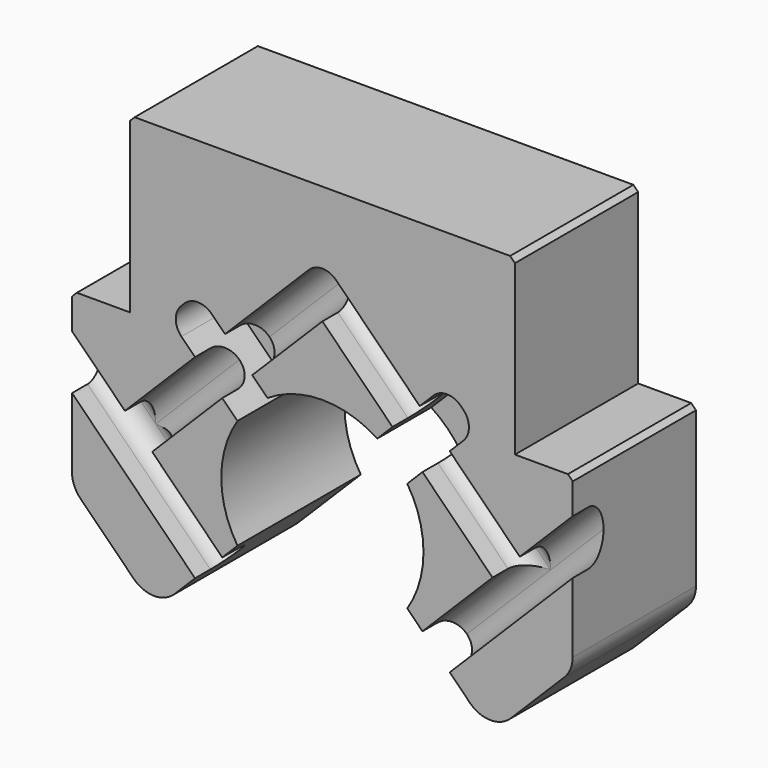
from build123d import *

# Parameters (mm, degrees)
F1_DEPTH = 16
F2_DEPTH = 7
F3_DEPTH = 4
F4_R     = 2
F5_R     = 1.9999
F6_R     = 3
F7_SIZE  = 0.5


# Not quite as in the source:
# - a fillet or chamfer is up to 0.001 mm smaller than in the source, because OpenCascade refuses the exact size
# - a feature names something its author has since deleted; it is built from what else it names


with BuildPart() as f1:
    # F0 (on Front) → F1 (new body)
    with BuildSketch(Plane.XZ):
        with BuildLine():
            ThreePointArc((-5.7041860158, 8.815455853), (0, 10.5), (5.7041860158, 8.815455853))
            Line((5.7041860158, 8.815455853), (7.2831998462, 10.3944696834))
            Line((7.2831998462, 10.3944696834), (0, 17.6776695297))
            Line((0, 17.6776695297), (-7.2831998462, 10.3944696834))
            Line((-7.2831998462, 10.3944696834), (-5.7041860158, 8.815455853))
        make_face()
        with BuildLine():
            ThreePointArc((-8.815455853, 5.7041860158), (-7.4246212025, 7.4246212025), (-5.7041860158, 8.815455853))
            Line((-5.7041860158, 8.815455853), (-7.2831998462, 10.3944696834))
            Line((-7.2831998462, 10.3944696834), (-10.3944696834, 7.2831998462))
            Line((-10.3944696834, 7.2831998462), (-8.815455853, 5.7041860158))
        make_face()
        with BuildLine():
            ThreePointArc((-8.815455853, -5.7041860158), (-10.5, 0), (-8.815455853, 5.7041860158))
            Line((-8.815455853, 5.7041860158), (-10.3944696834, 7.2831998462))
            Line((-10.3944696834, 7.2831998462), (-17.6776695297, 0))
            Line((-17.6776695297, 0), (-10.3944696834, -7.2831998462))
            Line((-10.3944696834, -7.2831998462), (-8.815455853, -5.7041860158))
        make_face()
        with BuildLine():
            ThreePointArc((5.7041860158, 8.815455853), (7.4246212025, 7.4246212025), (8.815455853, 5.7041860158))
            Line((8.815455853, 5.7041860158), (10.3944696834, 7.2831998462))
            Line((10.3944696834, 7.2831998462), (7.2831998462, 10.3944696834))
            Line((7.2831998462, 10.3944696834), (5.7041860158, 8.815455853))
        make_face()
        Polygon((0, 17.6776695297), (7.2831998462, 10.3944696834), (10.111626971, 13.2228968082), (0, 23.3345237792), (-10.111626971, 13.2228968082), (-7.2831998462, 10.3944696834), align=None)
        Polygon((7.2831998462, 10.3944696834), (10.3944696834, 7.2831998462), (13.2228968082, 10.111626971), (10.111626971, 13.2228968082), align=None)
        Polygon((-10.3944696834, 7.2831998462), (-7.2831998462, 10.3944696834), (-10.111626971, 13.2228968082), (-13.2228968082, 10.111626971), align=None)
        Polygon((-17.6776695297, 0), (-10.3944696834, 7.2831998462), (-13.2228968082, 10.111626971), (-20.5060966544, 2.8284271247), (-26, 8.3223304703), (-26, 2.6654762208), (-13.2228968082, -10.111626971), (-10.3944696834, -7.2831998462), align=None)
        Polygon((-13.2228968082, 10.111626971), (-10.111626971, 13.2228968082), (-12.9400540957, 16.0513239329), (-16.0513239329, 12.9400540957), align=None)
        Polygon((17.6776695297, 0), (10.3944696834, -7.2831998462), (13.2228968082, -10.111626971), (26, 2.6654762208), (26, 8.3223304703), (20.5060966544, 2.8284271247), (13.2228968082, 10.111626971), (10.3944696834, 7.2831998462), align=None)
        with BuildLine():
            ThreePointArc((8.815455853, 5.7041860158), (10.5, 0), (8.815455853, -5.7041860158))
            Line((8.815455853, -5.7041860158), (10.3944696834, -7.2831998462))
            Line((10.3944696834, -7.2831998462), (17.6776695297, 0))
            Line((17.6776695297, 0), (10.3944696834, 7.2831998462))
            Line((10.3944696834, 7.2831998462), (8.815455853, 5.7041860158))
        make_face()
        Polygon((16.0513239329, 12.9400540957), (13.2228968082, 10.111626971), (20.5060966544, 2.8284271247), (26, 8.3223304703), (26, 12), (20, 12), (20, 30), (0, 30), (-20, 30), (-20, 12), (-26, 12), (-26, 8.3223304703), (-20.5060966544, 2.8284271247), (-13.2228968082, 10.111626971), (-16.0513239329, 12.9400540957), (-12.9400540957, 16.0513239329), (-10.111626971, 13.2228968082), (0, 23.3345237792), (10.111626971, 13.2228968082), (12.9400540957, 16.0513239329), align=None)
        Polygon((10.111626971, 13.2228968082), (13.2228968082, 10.111626971), (16.0513239329, 12.9400540957), (12.9400540957, 16.0513239329), align=None)
        Polygon((26, 2.6654762208), (13.2228968082, -10.111626971), (17.4655374953, -14.3542676581), (26, -5.8198051534), align=None)
        Polygon((-17.4655374953, -14.3542676581), (-13.2228968082, -10.111626971), (-26, 2.6654762208), (-26, -5.8198051534), align=None)
    extrude(amount=-F1_DEPTH)

    # F0 (on Front) → F2 (cut)
    with BuildSketch(Plane.XZ):
        Polygon((10.111626971, 13.2228968082), (13.2228968082, 10.111626971), (16.0513239329, 12.9400540957), (12.9400540957, 16.0513239329), align=None)
        Polygon((7.2831998462, 10.3944696834), (10.3944696834, 7.2831998462), (13.2228968082, 10.111626971), (10.111626971, 13.2228968082), align=None)
        with BuildLine():
            ThreePointArc((5.7041860158, 8.815455853), (7.4246212025, 7.4246212025), (8.815455853, 5.7041860158))
            Line((8.815455853, 5.7041860158), (10.3944696834, 7.2831998462))
            Line((10.3944696834, 7.2831998462), (7.2831998462, 10.3944696834))
            Line((7.2831998462, 10.3944696834), (5.7041860158, 8.815455853))
        make_face()
        with BuildLine():
            ThreePointArc((-8.815455853, 5.7041860158), (-7.4246212025, 7.4246212025), (-5.7041860158, 8.815455853))
            Line((-5.7041860158, 8.815455853), (-7.2831998462, 10.3944696834))
            Line((-7.2831998462, 10.3944696834), (-10.3944696834, 7.2831998462))
            Line((-10.3944696834, 7.2831998462), (-8.815455853, 5.7041860158))
        make_face()
        Polygon((-13.2228968082, 10.111626971), (-10.111626971, 13.2228968082), (-12.9400540957, 16.0513239329), (-16.0513239329, 12.9400540957), align=None)
        Polygon((-10.3944696834, 7.2831998462), (-7.2831998462, 10.3944696834), (-10.111626971, 13.2228968082), (-13.2228968082, 10.111626971), align=None)
    extrude(amount=-F2_DEPTH, mode=Mode.SUBTRACT)

    # F0 (on Front) → F3 (cut)
    with BuildSketch(Plane.XZ):
        Polygon((0, 17.6776695297), (7.2831998462, 10.3944696834), (10.111626971, 13.2228968082), (0, 23.3345237792), (-10.111626971, 13.2228968082), (-7.2831998462, 10.3944696834), align=None)
        Polygon((17.6776695297, 0), (10.3944696834, -7.2831998462), (13.2228968082, -10.111626971), (26, 2.6654762208), (26, 8.3223304703), (20.5060966544, 2.8284271247), (13.2228968082, 10.111626971), (10.3944696834, 7.2831998462), align=None)
        Polygon((-17.6776695297, 0), (-10.3944696834, 7.2831998462), (-13.2228968082, 10.111626971), (-20.5060966544, 2.8284271247), (-26, 8.3223304703), (-26, 2.6654762208), (-13.2228968082, -10.111626971), (-10.3944696834, -7.2831998462), align=None)
    extrude(amount=-F3_DEPTH, mode=Mode.SUBTRACT)

    # F4
    f4_edges = [f1.edges().sort_by_distance(p)[0] for p in [
        (-16.051324, 3.5, 12.940054),
        (-12.940054, 3.5, 16.051324),
        (12.940054, 3.5, 16.051324),
        (16.051324, 3.5, 12.940054),
        (0, 2, 23.334524),
    ]]
    fillet(f4_edges, radius=F4_R)

    # F5 (radius 2 in the source; OpenCascade refuses exactly that, so slightly less here)
    f5_edges = [f1.edges().sort_by_distance(p)[0] for p in [
        (19.611448, 4, -3.723075),
        (14.03607, 4, -3.6416),
        (14.03607, 4, 3.6416),
        (16.864497, 4, 6.470027),
        (5.76292, 4, 17.571604),
        (-16.864497, 4, 6.470027),
        (-23.253048, 4, 5.575379),
        (-14.03607, 4, -3.6416),
        (-3.6416, 4, 14.03607),
        (-14.03607, 4, 3.6416),
        (-19.611448, 4, -3.723075),
        (23.253048, 4, 5.575379),
        (0, 4, 22.506097),
        (-5.76292, 4, 17.571604),
        (3.6416, 4, 14.03607),
    ]]
    fillet(f5_edges, radius=F5_R)

    # F6
    f6_edges = [f1.edges().sort_by_distance(p)[0] for p in [
        (17.465537, 8, -14.354268),
        (26, 8, -5.819805),
        (-26, 8, -5.819805),
        (-17.465537, 8, -14.354268),
    ]]
    fillet(f6_edges, radius=F6_R)

    # F7
    f7_edges = [f1.edges().sort_by_distance(p)[0] for p in [
        (20, 8, 30),
        (26, 8, 12),
        (-20, 8, 30),
        (-26, 8, 12),
    ]]
    chamfer(f7_edges, length=F7_SIZE)


solid = f1.part
